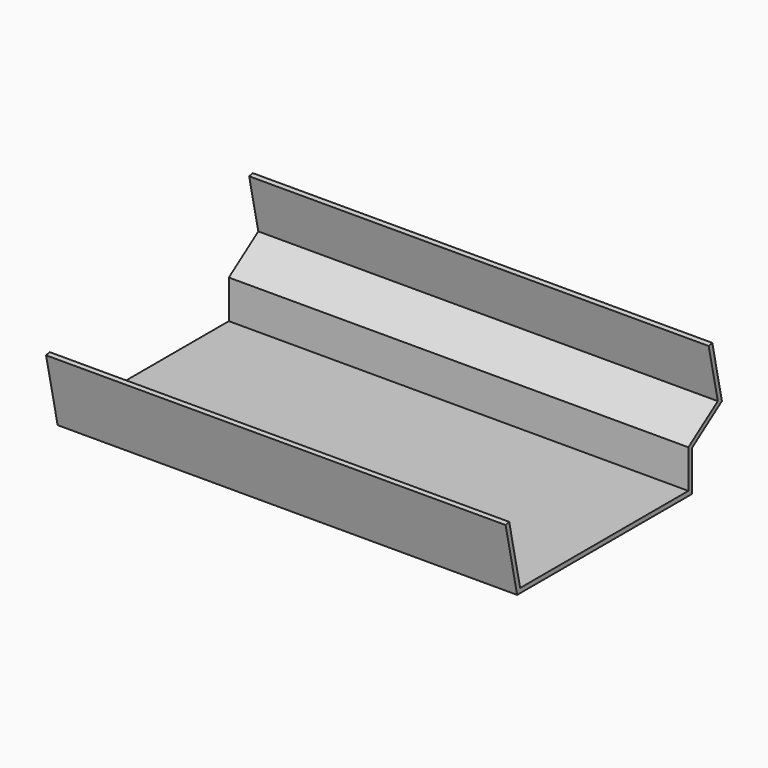
from build123d import *

# Parameters (mm, degrees)
F1_DEPTH = 400


# Not quite as in the source:
# - a feature names something its author has since deleted; it is built from what else it names


with BuildPart() as f1:
    # F0 (on Right) → F1 (new body)
    with BuildSketch(Plane.YZ):
        Polygon((-62.5913035921, 0.8380515879), (-66.5025271265, 0), (-53.9317533084, -58.668353016), (136.3489470076, -58.668353016), (136.3489470076, -23.3414838178), (168.86847095, -0.7023278775), (158.3928261017, 48.1879663026), (154.4816025673, 47.3499147147), (164.3999275858, 1.060656636), (132.3489470076, -21.2523129091), (132.3489470076, -54.668353016), (-50.6980353843, -54.668353016), align=None)
    extrude(amount=F1_DEPTH)


solid = f1.part
